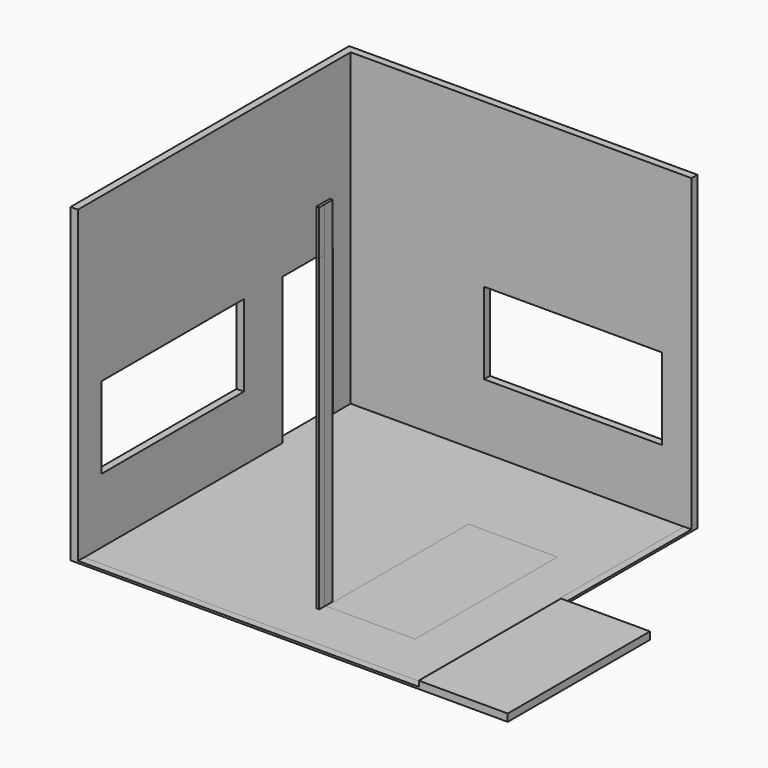
from build123d import *

# Parameters (mm, degrees)
F0_W      = 19.05
F0_H      = 63.5
F1_DEPTH  = 2438.4
F0_H_2    = 25.4
F2_DEPTH  = 2438.4
F3_DEPTH  = 2438.4
F4_DEPTH  = 2438.4
F5_DEPTH  = 914.4
F6_DEPTH  = 1219.2
F7_DEPTH  = 1828.8
F8_DEPTH  = 609.6
F9_DEPTH  = 1828.8
F10_DEPTH = 1219.2
F11_DEPTH = 914.4
F12_DEPTH = 609.6
F13_DEPTH = 762
F14_DEPTH = 1828.8
F15_W     = 101.6
F15_H     = 863.6
F16_DEPTH = 25.4
F15_W_2   = 1219.2
F15_H_2   = 2438.4
F17_DEPTH = 6.35
F15_H_3   = 660.4
F18_DEPTH = 4267.2
F19_DEPTH = 27.94
F20_START = 2032
F15_W_3   = 2438.4
F15_H_4   = 101.6
F20_DEPTH = 2235.2
F21_DEPTH = 914.4
F22_DEPTH = 101.6
F23_DEPTH = 2352.675
F24_DEPTH = 4267.2
F25_DEPTH = 4876.8
F26_DEPTH = 254
F27_DEPTH = 101.6
F28_DEPTH = 4876.8
F29_DEPTH = 4267.2
F30_W     = 609.6
F30_H     = 2438.4
F31_DEPTH = 25.4
F32_DEPTH = 25.4


with BuildPart() as f1:
    # F0 (on Top) → F1 (new body)
    with BuildSketch(Plane.XY):
        with Locations((-42.2796816051, 120.7831952572)):
            Rectangle(F0_W, F0_H)
    extrude(amount=F1_DEPTH)


with BuildPart() as f2:
    # F0 (on Top) → F2 (new body)
    with BuildSketch(Plane.XY):
        with Locations((-42.2796816051, 120.7831952572)):
            Rectangle(F0_W, F0_H)
        with Locations((-42.2796816051, 76.3331952572)):
            Rectangle(F0_W, F0_H_2)
    extrude(amount=F2_DEPTH)


with BuildPart() as f3:
    # F0 (on Top) → F3 (new body)
    with BuildSketch(Plane.XY):
        with Locations((-42.2796816051, 120.7831952572)):
            Rectangle(F0_W, F0_H)
        with Locations((-23.2296816051, 120.7831952572)):
            Rectangle(F0_W, F0_H)
    extrude(amount=F3_DEPTH)


with BuildPart() as f4:
    # F0 (on Top) → F4 (new body)
    with BuildSketch(Plane.XY):
        with Locations((-42.2796816051, 120.7831952572)):
            Rectangle(F0_W, F0_H)
        with Locations((-23.2296816051, 120.7831952572)):
            Rectangle(F0_W, F0_H)
        with Locations((-42.2796816051, 76.3331952572)):
            Rectangle(F0_W, F0_H_2)
        with Locations((-23.2296816051, 76.3331952572)):
            Rectangle(F0_W, F0_H_2)
    extrude(amount=F4_DEPTH)


with BuildPart() as f5:
    # F0 (on Top) → F5 (new body)
    with BuildSketch(Plane.XY):
        with Locations((-42.2796816051, 120.7831952572)):
            Rectangle(F0_W, F0_H)
        with Locations((-23.2296816051, 120.7831952572)):
            Rectangle(F0_W, F0_H)
        with Locations((-23.2296816051, 76.3331952572)):
            Rectangle(F0_W, F0_H_2)
        with Locations((-42.2796816051, 76.3331952572)):
            Rectangle(F0_W, F0_H_2)
    extrude(amount=F5_DEPTH)


with BuildPart() as f6:
    # F0 (on Top) → F6 (new body)
    with BuildSketch(Plane.XY):
        with Locations((-42.2796816051, 120.7831952572)):
            Rectangle(F0_W, F0_H)
        with Locations((-23.2296816051, 120.7831952572)):
            Rectangle(F0_W, F0_H)
        with Locations((-23.2296816051, 76.3331952572)):
            Rectangle(F0_W, F0_H_2)
        with Locations((-42.2796816051, 76.3331952572)):
            Rectangle(F0_W, F0_H_2)
    extrude(amount=F6_DEPTH)


with BuildPart() as f7:
    # F0 (on Top) → F7 (new body)
    with BuildSketch(Plane.XY):
        with Locations((-42.2796816051, 120.7831952572)):
            Rectangle(F0_W, F0_H)
        with Locations((-23.2296816051, 120.7831952572)):
            Rectangle(F0_W, F0_H)
        with Locations((-23.2296816051, 76.3331952572)):
            Rectangle(F0_W, F0_H_2)
        with Locations((-42.2796816051, 76.3331952572)):
            Rectangle(F0_W, F0_H_2)
    extrude(amount=F7_DEPTH)


with BuildPart() as f8:
    # F0 (on Top) → F8 (new body)
    with BuildSketch(Plane.XY):
        with Locations((-42.2796816051, 120.7831952572)):
            Rectangle(F0_W, F0_H)
        with Locations((-23.2296816051, 120.7831952572)):
            Rectangle(F0_W, F0_H)
        with Locations((-23.2296816051, 76.3331952572)):
            Rectangle(F0_W, F0_H_2)
        with Locations((-42.2796816051, 76.3331952572)):
            Rectangle(F0_W, F0_H_2)
    extrude(amount=F8_DEPTH)


with BuildPart() as f9:
    # F0 (on Top) → F9 (new body)
    with BuildSketch(Plane.XY):
        with Locations((-42.2796816051, 120.7831952572)):
            Rectangle(F0_W, F0_H)
        with Locations((-23.2296816051, 120.7831952572)):
            Rectangle(F0_W, F0_H)
    extrude(amount=F9_DEPTH)


with BuildPart() as f10:
    # F0 (on Top) → F10 (new body)
    with BuildSketch(Plane.XY):
        with Locations((-42.2796816051, 120.7831952572)):
            Rectangle(F0_W, F0_H)
        with Locations((-23.2296816051, 120.7831952572)):
            Rectangle(F0_W, F0_H)
    extrude(amount=F10_DEPTH)


with BuildPart() as f11:
    # F0 (on Top) → F11 (new body)
    with BuildSketch(Plane.XY):
        with Locations((-42.2796816051, 120.7831952572)):
            Rectangle(F0_W, F0_H)
        with Locations((-23.2296816051, 120.7831952572)):
            Rectangle(F0_W, F0_H)
    extrude(amount=F11_DEPTH)


with BuildPart() as f12:
    # F0 (on Top) → F12 (new body)
    with BuildSketch(Plane.XY):
        with Locations((-42.2796816051, 120.7831952572)):
            Rectangle(F0_W, F0_H)
        with Locations((-23.2296816051, 120.7831952572)):
            Rectangle(F0_W, F0_H)
    extrude(amount=F12_DEPTH)


with BuildPart() as f13:
    # F0 (on Top) → F13 (new body)
    with BuildSketch(Plane.XY):
        with Locations((-42.2796816051, 120.7831952572)):
            Rectangle(F0_W, F0_H)
        with Locations((-23.2296816051, 120.7831952572)):
            Rectangle(F0_W, F0_H)
    extrude(amount=F13_DEPTH)


with BuildPart() as f14:
    # F0 (on Top) → F14 (new body)
    with BuildSketch(Plane.XY):
        with Locations((-23.2296816051, 76.3331952572)):
            Rectangle(F0_W, F0_H_2)
        with Locations((-42.2796816051, 76.3331952572)):
            Rectangle(F0_W, F0_H_2)
    extrude(amount=F14_DEPTH)


with BuildPart() as f16:
    # F15 (on Top) → F16 (new body)
    with BuildSketch(Plane.XY):
        Polygon((-901.7698979378, 3997.985077095), (-2730.5698979378, 3997.985077095), (-2730.5698979378, 3693.185077095), (-2730.5698979378, 2829.585077095), (-2730.5698979378, 2169.185077095), (-2730.5698979378, -269.214922905), (-2730.5698979378, -574.014922905), (1841.4301020622, -574.014922905), (1841.4301020622, 3997.985077095), (1536.6301020622, 3997.985077095), align=None)
        with Locations((-2781.3698979378, 3261.385077095)):
            Rectangle(F15_W, F15_H)
    extrude(amount=F16_DEPTH)

    # F15 (on Top) → F18 (join)
    with BuildSketch(Plane.XY):
        with Locations((-2781.3698979378, 2499.385077095)):
            Rectangle(F15_W, F15_H_3)
        Polygon((1536.6301020622, 4099.585077095), (1536.6301020622, 3997.985077095), (1841.4301020622, 3997.985077095), (1943.0301020622, 3997.985077095), (1943.0301020622, 4099.585077095), align=None)
        Polygon((-2730.5698979378, 3693.185077095), (-2730.5698979378, 3997.985077095), (-901.7698979378, 3997.985077095), (-901.7698979378, 4099.585077095), (-2832.1698979378, 4099.585077095), (-2832.1698979378, 3693.185077095), align=None)
        Polygon((-2730.5698979378, -574.014922905), (-2730.5698979378, -269.214922905), (-2832.1698979378, -269.214922905), (-2832.1698979378, -675.614922905), (-2730.5698979378, -675.614922905), align=None)
    extrude(amount=F18_DEPTH)

    # F15 (on Top) → F19 (join)
    with BuildSketch(Plane.XY):
        Polygon((1943.0301020622, 3997.985077095), (1841.4301020622, 3997.985077095), (1841.4301020622, -574.014922905), (-2730.5698979378, -574.014922905), (-2730.5698979378, -675.614922905), (1943.0301020622, -675.614922905), (1943.0301020622, 1762.785077095), align=None)
    extrude(amount=F19_DEPTH)

    # F15 (on Top) → F20 (join)
    with BuildSketch(Plane.XY.offset(F20_START)):
        with Locations((-2781.3698979378, 3261.385077095)):
            Rectangle(F15_W, F15_H)
        with Locations((-2781.3698979378, 949.985077095)):
            Rectangle(F15_W, F15_H_2)
        with Locations((317.4301020622, 4048.785077095)):
            Rectangle(F15_W_3, F15_H_4)
    extrude(amount=F20_DEPTH)

    # F15 (on Top) → F21 (join)
    with BuildSketch(Plane.XY):
        with Locations((-2781.3698979378, 949.985077095)):
            Rectangle(F15_W, F15_H_2)
        with Locations((317.4301020622, 4048.785077095)):
            Rectangle(F15_W_3, F15_H_4)
    extrude(amount=F21_DEPTH)


with BuildPart() as f17:
    # F15 (on Top) → F17 (new body)
    with BuildSketch(Plane.XY):
        with Locations((2552.6301020622, 543.585077095)):
            Rectangle(F15_W_2, F15_H_2)
    extrude(amount=F17_DEPTH)


with BuildPart() as f22:
    # F15 (on Top) → F22 (new body)
    with BuildSketch(Plane.XY):
        with Locations((2552.6301020622, 543.585077095)):
            Rectangle(F15_W_2, F15_H_2)
    extrude(amount=F22_DEPTH)


with BuildPart() as f23:
    # F0 (on Top) → F23 (new body)
    with BuildSketch(Plane.XY):
        with Locations((-42.2796816051, 120.7831952572)):
            Rectangle(F0_W, F0_H)
        with Locations((-23.2296816051, 120.7831952572)):
            Rectangle(F0_W, F0_H)
        with Locations((-42.2796816051, 76.3331952572)):
            Rectangle(F0_W, F0_H_2)
        with Locations((-23.2296816051, 76.3331952572)):
            Rectangle(F0_W, F0_H_2)
    extrude(amount=F23_DEPTH)


with BuildPart() as f24:
    # F0 (on Top) → F24 (new body)
    with BuildSketch(Plane.XY):
        Polygon((-51.8046816051, 292.2331952572), (-51.8046816051, 152.5331952572), (-32.7546816051, 152.5331952572), (-13.7046816051, 152.5331952572), (-13.7046816051, 292.2331952572), align=None)
    extrude(amount=F24_DEPTH)


with BuildPart() as f25:
    # F0 (on Top) → F25 (new body)
    with BuildSketch(Plane.XY):
        Polygon((-51.8046816051, 292.2331952572), (-51.8046816051, 152.5331952572), (-32.7546816051, 152.5331952572), (-13.7046816051, 152.5331952572), (-13.7046816051, 292.2331952572), align=None)
    extrude(amount=F25_DEPTH)


with BuildPart() as f26:
    # F0 (on Top) → F26 (new body)
    with BuildSketch(Plane.XY):
        with Locations((-42.2796816051, 76.3331952572)):
            Rectangle(F0_W, F0_H_2)
        with Locations((-42.2796816051, 120.7831952572)):
            Rectangle(F0_W, F0_H)
        with Locations((-23.2296816051, 120.7831952572)):
            Rectangle(F0_W, F0_H)
        with Locations((-23.2296816051, 76.3331952572)):
            Rectangle(F0_W, F0_H_2)
    extrude(amount=F26_DEPTH)


with BuildPart() as f27:
    # F0 (on Top) → F27 (new body)
    with BuildSketch(Plane.XY):
        with Locations((-42.2796816051, 76.3331952572)):
            Rectangle(F0_W, F0_H_2)
        with Locations((-42.2796816051, 120.7831952572)):
            Rectangle(F0_W, F0_H)
        with Locations((-23.2296816051, 120.7831952572)):
            Rectangle(F0_W, F0_H)
        with Locations((-23.2296816051, 76.3331952572)):
            Rectangle(F0_W, F0_H_2)
    extrude(amount=F27_DEPTH)


with BuildPart() as f28:
    # F0 (on Top) → F28 (new body)
    with BuildSketch(Plane.XY):
        with Locations((-42.2796816051, 76.3331952572)):
            Rectangle(F0_W, F0_H_2)
        with Locations((-42.2796816051, 120.7831952572)):
            Rectangle(F0_W, F0_H)
        with Locations((-23.2296816051, 120.7831952572)):
            Rectangle(F0_W, F0_H)
        with Locations((-23.2296816051, 76.3331952572)):
            Rectangle(F0_W, F0_H_2)
    extrude(amount=F28_DEPTH)


with BuildPart() as f29:
    # F0 (on Top) → F29 (new body)
    with BuildSketch(Plane.XY):
        with Locations((-42.2796816051, 120.7831952572)):
            Rectangle(F0_W, F0_H)
        with Locations((-23.2296816051, 120.7831952572)):
            Rectangle(F0_W, F0_H)
        with Locations((-23.2296816051, 76.3331952572)):
            Rectangle(F0_W, F0_H_2)
        with Locations((-42.2796816051, 76.3331952572)):
            Rectangle(F0_W, F0_H_2)
    extrude(amount=F29_DEPTH)


with BuildPart() as f31:
    # F30 (on Top) → F31 (new body)
    with BuildSketch(Plane.XY):
        with Locations((304.8, 1385.8409522295)):
            Rectangle(F30_W, F30_H)
    extrude(amount=F31_DEPTH)


with BuildPart() as f32:
    # F30 (on Top) → F32 (new body)
    with BuildSketch(Plane.XY):
        with Locations((304.8, 1385.8409522295)):
            Rectangle(F30_W, F30_H)
        with Locations((914.4, 1385.8409522295)):
            Rectangle(F30_W, F30_H)
    extrude(amount=F32_DEPTH)


solid = Compound([f1.part, f2.part, f3.part, f4.part, f5.part, f6.part, f7.part, f8.part, f9.part, f10.part, f11.part, f12.part, f13.part, f14.part, f16.part, f17.part, f22.part, f23.part, f24.part, f25.part, f26.part, f27.part, f28.part, f29.part, f31.part, f32.part])
